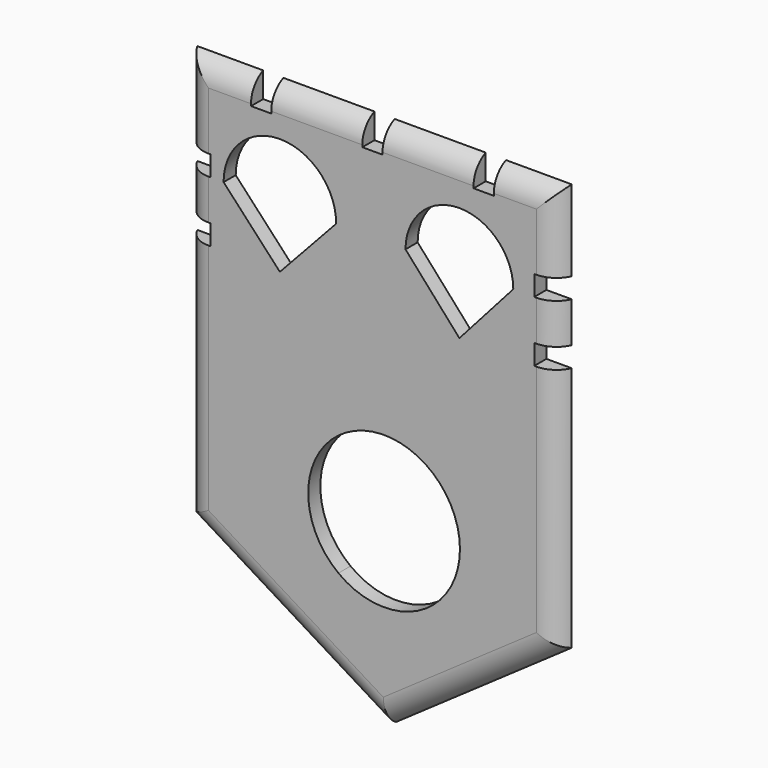
from build123d import *

# Parameters (mm, degrees)
F1_DEPTH     = 3
F2_T1_DEPTH  = 69.0608621697
F2_T3_DEPTH  = 65.2081986538
F2_T5_DEPTH  = 71.5756555765
F2_T7_DEPTH  = 30.9128784748
F2_T9_DEPTH  = 38.9128784748
F2_T11_DEPTH = 35.9128784748
F2_T13_DEPTH = 40.9128784748
F2_T15_DEPTH = 40.9128784748
F2_T17_DEPTH = 35.9128784748


# Not quite as in the source:
# - a fillet or chamfer that OpenCascade refuses, or shapes differently, is made with other operations: its cross-section is extruded or revolved along the edge and cut away or added


with BuildPart() as f1:
    # F0 (on Front) → F1 (new body)
    with BuildSketch(Plane.XZ):
        with BuildLine():
            Line((-39.3023127707, 0), (-39.3023127707, -40.6627771018))
            Line((-39.3023127707, -40.6627771018), (-9.0223597329, -40.6627771018))
            ThreePointArc((-9.0223597329, -40.6627771018), (-6.6956927949, -15.256923351), (15, -28.6795794964))
            ThreePointArc((15, -28.6795794964), (13.4226561454, -35.3752722912), (9.0223597329, -40.6627771018))
            Line((9.0223597329, -40.6627771018), (34.6976872293, -40.6627771018))
            Line((34.6976872293, -40.6627771018), (34.6976872293, 0))
            Line((34.6976872293, 0), (34.6976872293, 8))
            Line((34.6976872293, 8), (29.6976872293, 8))
            Line((29.6976872293, 8), (29.6976872293, 12))
            Line((29.6976872293, 12), (34.6976872293, 12))
            Line((34.6976872293, 12), (34.6976872293, 20))
            Line((34.6976872293, 20), (29.6976872293, 20))
            Line((29.6976872293, 20), (29.6976872293, 24))
            Line((29.6976872293, 24), (34.6976872293, 24))
            Line((34.6976872293, 24), (34.6976872293, 40))
            Line((34.6976872293, 40), (21.6976872293, 40))
            Line((21.6976872293, 40), (21.6976872293, 35))
            Line((21.6976872293, 35), (17.6976872293, 35))
            Line((17.6976872293, 35), (17.6976872293, 40))
            Line((17.6976872293, 40), (-0.3023127707, 40))
            Line((-0.3023127707, 40), (-0.3023127707, 35))
            Line((-0.3023127707, 35), (-4.3023127707, 35))
            Line((-4.3023127707, 35), (-4.3023127707, 40))
            Line((-4.3023127707, 40), (-22.3023127707, 40))
            Line((-22.3023127707, 40), (-22.3023127707, 35))
            Line((-22.3023127707, 35), (-26.3023127707, 35))
            Line((-26.3023127707, 35), (-26.3023127707, 40))
            Line((-26.3023127707, 40), (-39.3023127707, 40))
            Line((-39.3023127707, 40), (-39.3023127707, 24))
            Line((-39.3023127707, 24), (-34.3023127707, 24))
            Line((-34.3023127707, 24), (-34.3023127707, 20))
            Line((-34.3023127707, 20), (-39.3023127707, 20))
            Line((-39.3023127707, 20), (-39.3023127707, 12))
            Line((-39.3023127707, 12), (-34.3023127707, 12))
            Line((-34.3023127707, 12), (-34.3023127707, 8))
            Line((-34.3023127707, 8), (-39.3023127707, 8))
            Line((-39.3023127707, 8), (-39.3023127707, 0))
        make_face()
        with BuildLine():
            ThreePointArc((-31.7284863554, 20), (-20.5985922366, 31.1298941188), (-9.4686981178, 20))
            Line((-9.4686981178, 20), (-20.5985922366, 8))
            Line((-20.5985922366, 8), (-31.7284863554, 20))
        make_face(mode=Mode.SUBTRACT)
        with BuildLine():
            ThreePointArc((4.2398196727, 20), (14.8943690583, 30.6545493856), (25.5489184439, 20))
            Line((25.5489184439, 20), (14.8943690583, 8))
            Line((14.8943690583, 8), (4.2398196727, 20))
        make_face(mode=Mode.SUBTRACT)
        with BuildLine():
            Line((-9.0223597329, -40.6627771018), (-39.3023127707, -40.6627771018))
            Line((-39.3023127707, -40.6627771018), (0, -64.8488187371))
            Line((0, -64.8488187371), (34.6976872293, -40.6627771018))
            Line((34.6976872293, -40.6627771018), (9.0223597329, -40.6627771018))
            ThreePointArc((9.0223597329, -40.6627771018), (0, -43.6795794964), (-9.0223597329, -40.6627771018))
        make_face()
    extrude(amount=F1_DEPTH)

    # F2: fillet of radius 5 on 12 edges, made by hand

    # F2_s2 → F2_t1 (cut)
    with BuildSketch(Plane(origin=(-20.1138870842, 0, 12.3777782062), x_dir=(0, 1, 0), z_dir=(0.8516582876, 0, -0.5240974729))):
        with BuildLine():
            ThreePointArc((0, -55.2290339197), (-2.1833001327, -53.3850710123), (-3, -50.6464582247))
            Line((-3, -50.6464582247), (-3, -55.2290339197))
            Line((-3, -55.2290339197), (0, -55.2290339197))
        make_face()
    extrude(amount=F2_T1_DEPTH, mode=Mode.SUBTRACT)

    # F2_s4 → F2_t3 (cut)
    with BuildSketch(Plane(origin=(-39.8201349052, 0, -27.7566465561), x_dir=(0, 1, 0), z_dir=(0.8203670544, 0, 0.5718372986))):
        with BuildLine():
            ThreePointArc((0, -53.1998344073), (-2.1833001327, -51.3558714999), (-3, -48.6172587124))
            Line((-3, -48.6172587124), (-3, -53.1998344073))
            Line((-3, -53.1998344073), (0, -53.1998344073))
        make_face()
    extrude(amount=F2_T3_DEPTH, mode=Mode.SUBTRACT)

    # F2_s6 → F2_t5 (cut)
    with BuildSketch(Plane.XY.offset(-52.1192163392)):
        with BuildLine():
            ThreePointArc((-39.3023127707, 0), (-37.4583498632, -2.1833001327), (-34.7197370757, -3))
            Line((-34.7197370757, -3), (-39.3023127707, -3))
            Line((-39.3023127707, -3), (-39.3023127707, 0))
        make_face()
        with BuildLine():
            ThreePointArc((34.6976872293, 0), (32.8537243219, -2.1833001327), (30.1151115344, -3))
            Line((30.1151115344, -3), (34.6976872293, -3))
            Line((34.6976872293, -3), (34.6976872293, 0))
        make_face()
    extrude(amount=F2_T5_DEPTH, mode=Mode.SUBTRACT)

    # F2_s8 → F2_t7 (cut)
    with BuildSketch(Plane.XY.offset(0.5435607626)):
        with BuildLine():
            ThreePointArc((-39.3023127707, 0), (-37.4583498632, -2.1833001327), (-34.7197370757, -3))
            Line((-34.7197370757, -3), (-39.3023127707, -3))
            Line((-39.3023127707, -3), (-39.3023127707, 0))
        make_face()
        with BuildLine():
            ThreePointArc((34.6976872293, 0), (32.8537243219, -2.1833001327), (30.1151115344, -3))
            Line((30.1151115344, -3), (34.6976872293, -3))
            Line((34.6976872293, -3), (34.6976872293, 0))
        make_face()
    extrude(amount=F2_T7_DEPTH, mode=Mode.SUBTRACT)

    # F2_s10 → F2_t9 (cut)
    with BuildSketch(Plane.XY.offset(12.5435607626)):
        with BuildLine():
            ThreePointArc((-39.3023127707, 0), (-37.4583498632, -2.1833001327), (-34.7197370757, -3))
            Line((-34.7197370757, -3), (-39.3023127707, -3))
            Line((-39.3023127707, -3), (-39.3023127707, 0))
        make_face()
        with BuildLine():
            ThreePointArc((34.6976872293, 0), (32.8537243219, -2.1833001327), (30.1151115344, -3))
            Line((30.1151115344, -3), (34.6976872293, -3))
            Line((34.6976872293, -3), (34.6976872293, 0))
        make_face()
    extrude(amount=F2_T9_DEPTH, mode=Mode.SUBTRACT)

    # F2_s12 → F2_t11 (cut)
    with BuildSketch(Plane.YZ.offset(-50.7587520081)):
        with BuildLine():
            ThreePointArc((0, 40), (-2.1833001327, 38.1560370926), (-3, 35.417424305))
            Line((-3, 35.417424305), (-3, 40))
            Line((-3, 40), (0, 40))
        make_face()
    extrude(amount=F2_T11_DEPTH, mode=Mode.SUBTRACT)

    # F2_s14 → F2_t13 (cut)
    with BuildSketch(Plane.YZ.offset(-33.7587520081)):
        with BuildLine():
            ThreePointArc((0, 40), (-2.1833001327, 38.1560370926), (-3, 35.417424305))
            Line((-3, 35.417424305), (-3, 40))
            Line((-3, 40), (0, 40))
        make_face()
    extrude(amount=F2_T13_DEPTH, mode=Mode.SUBTRACT)

    # F2_s16 → F2_t15 (cut)
    with BuildSketch(Plane.YZ.offset(-11.7587520081)):
        with BuildLine():
            ThreePointArc((0, 40), (-2.1833001327, 38.1560370926), (-3, 35.417424305))
            Line((-3, 35.417424305), (-3, 40))
            Line((-3, 40), (0, 40))
        make_face()
    extrude(amount=F2_T15_DEPTH, mode=Mode.SUBTRACT)

    # F2_s18 → F2_t17 (cut)
    with BuildSketch(Plane.YZ.offset(10.2412479919)):
        with BuildLine():
            ThreePointArc((0, 40), (-2.1833001327, 38.1560370926), (-3, 35.417424305))
            Line((-3, 35.417424305), (-3, 40))
            Line((-3, 40), (0, 40))
        make_face()
    extrude(amount=F2_T17_DEPTH, mode=Mode.SUBTRACT)


solid = f1.part
